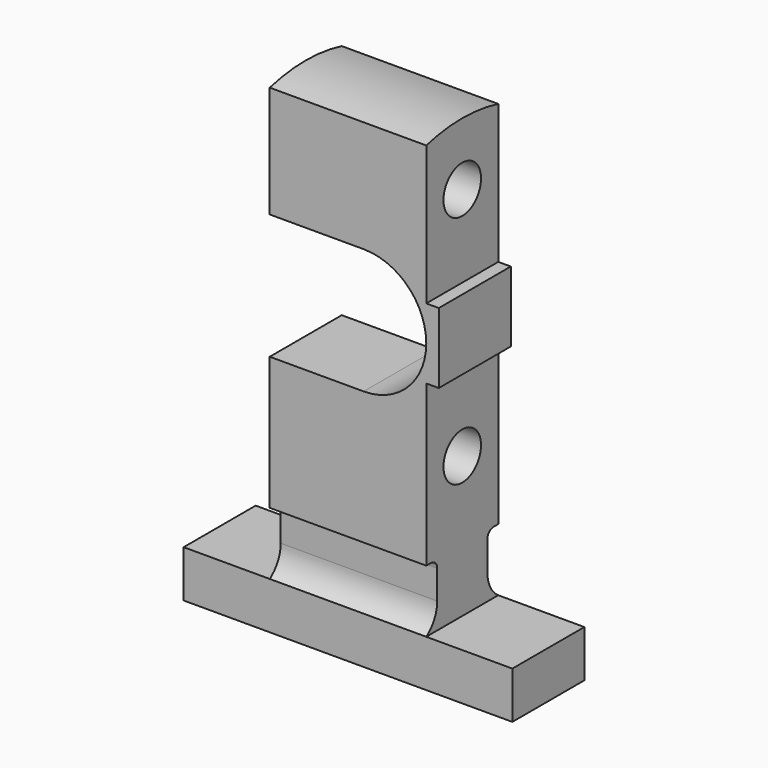
from build123d import *

# Parameters (mm, degrees)
F1_DEPTH      = 28.75
F3_DEPTH      = 105.001
F3_DEPTH_BACK = 105.001
F4_T1_DEPTH   = 100
F5_R          = 5
F7_D          = 30


# Not quite as in the source:
# - a fillet or chamfer that OpenCascade refuses, or shapes differently, is made with other operations: its cross-section is extruded or revolved along the edge and cut away or added


with BuildPart() as f1:
    # F0 (on Front) → F1 (new body, symmetric)
    with BuildSketch(Plane.XZ):
        with BuildLine():
            Line((-105, 30), (-105, 0))
            Line((-105, 0), (105, 0))
            Line((105, 0), (105, 30))
            Line((105, 30), (50, 30))
            Line((50, 30), (50, 172.5))
            Line((50, 172.5), (58, 172.5))
            Line((58, 172.5), (58, 217.5))
            Line((58, 217.5), (50, 217.5))
            Line((50, 217.5), (50, 315))
            Line((50, 315), (-50, 315))
            Line((-50, 315), (-50, 235))
            Line((-50, 235), (10, 235))
            ThreePointArc((10, 235), (50, 195), (10, 155))
            Line((10, 155), (-50, 155))
            Line((-50, 155), (-50, 30))
            Line((-50, 30), (-105, 30))
        make_face()
    extrude(amount=F1_DEPTH, both=True)

    # F2 (on Right) → F3 (cut, two sides)
    with BuildSketch(Plane.YZ) as f3_sk:
        with BuildLine():
            Line((-129.573866725, 348.6788272858), (-129.573866725, 30))
            Line((-129.573866725, 30), (-20, 30))
            Line((-20, 30), (-20, 70))
            Line((-20, 70), (-28.75, 70))
            Line((-28.75, 70), (-28.75, 306.3482712035))
            ThreePointArc((-28.75, 306.3482712035), (0, 310), (28.75, 306.3482712035))
            Line((28.75, 306.3482712035), (28.75, 70))
            Line((28.75, 70), (20, 70))
            Line((20, 70), (20, 30))
            Line((20, 30), (130.780075267, 30))
            Line((130.780075267, 30), (130.780075267, 348.6788272858))
            Line((130.780075267, 348.6788272858), (-129.573866725, 348.6788272858))
        make_face()
    extrude(amount=-F3_DEPTH, mode=Mode.SUBTRACT)
    extrude(f3_sk.sketch, amount=F3_DEPTH_BACK, mode=Mode.SUBTRACT)

    # F4: fillet of radius 20 on 2 edges, made by hand

    # F4_s2 → F4_t1 (join)
    with BuildSketch(Plane.YZ.offset(-50)):
        with BuildLine():
            ThreePointArc((-20, 46.5359456942), (-22.3223304703, 37.1818022272), (-28.75, 30))
            Line((-28.75, 30), (-20, 30))
            Line((-20, 30), (-20, 46.5359456942))
        make_face()
        with BuildLine():
            ThreePointArc((20, 46.5359456942), (22.3223304703, 37.1818022272), (28.75, 30))
            Line((28.75, 30), (20, 30))
            Line((20, 30), (20, 46.5359456942))
        make_face()
    extrude(amount=F4_T1_DEPTH)

    # F5
    f5_edges = [f1.edges().sort_by_distance(p)[0] for p in [
        (0, 20, 70),
        (0, -20, 70),
    ]]
    fillet(f5_edges, radius=F5_R)

    # F7 (through all)
    with Locations(Plane(origin=(-50, 0, 0), x_dir=(0, -1, 0), z_dir=(-1, 0, 0))):
        with Locations((0, 270), (0, 120)):
            Hole(F7_D / 2)


solid = f1.part
